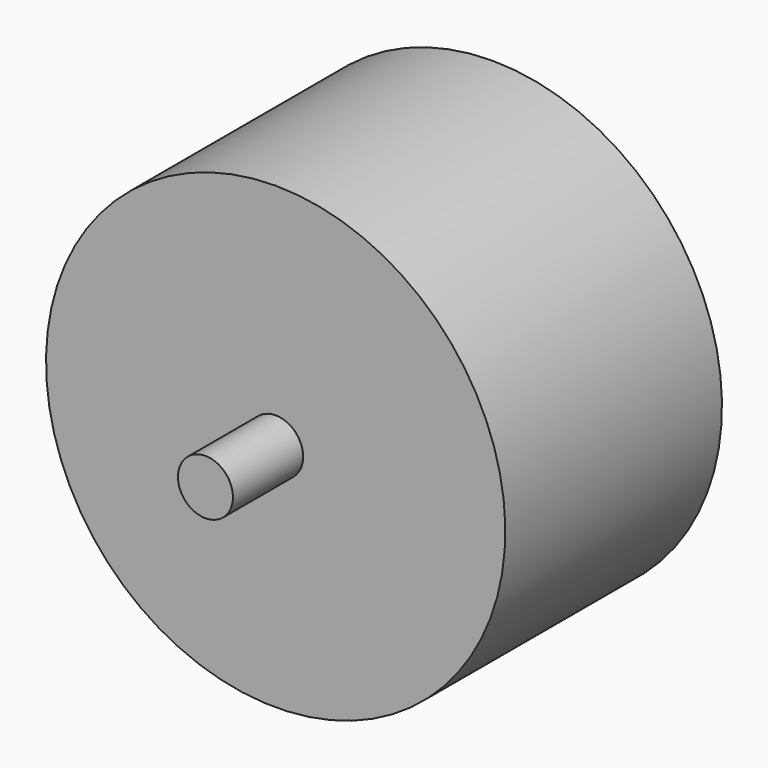
from build123d import *

# Parameters (mm, degrees)
F0_W         = 152.3266881704
F0_H         = 76.2925669551
F1_DEPTH     = 44.45
F2_T         = -2.54
F3_W         = 18.5941308737
F3_H         = 8.1849619746
F4_DEPTH     = 38.1
F5_T         = 2.54
F5_T3_DEPTH  = 13.2649619746
F5_T5_DEPTH  = 23.6741308737
F5_T7_DEPTH  = 78.8325669551
F5_T9_DEPTH  = 44.45
F5_T11_DEPTH = 152.3266881704
F7_R         = 5.6737308036
F8_DEPTH     = 89.211769402
F9_W         = 55.9205748141
F9_H         = 47.4143326283


# Not quite as in the source:
# - a shell that OpenCascade refuses in one call is made with other operations: the cavity is built on its own and cut out


with BuildPart() as f1:
    # F0 (on Front) → F1 (new body)
    with BuildSketch(Plane.XZ):
        with Locations((0.0222995877, 38.1462834775)):
            Rectangle(F0_W, F0_H)
    extrude(amount=F1_DEPTH)

    # F2
    f2_openings = [f1.faces().sort_by_distance(p)[0] for p in [
        (0.0223, -22.225, 0),
    ]]
    offset(amount=F2_T, openings=f2_openings)

    # F3 (on face) → F4 (join)
    with BuildSketch(Plane(origin=(-76.1410444975, 0, 0), x_dir=(0, -1, 0), z_dir=(-1, 0, 0))):
        with Locations((25.1720361412, 52.4518452585)):
            Rectangle(F3_W, F3_H)
    extrude(amount=F4_DEPTH)

    # F5: shell of thickness 2.54, made by hand


with BuildPart() as f5_core1:
    # F5_t2: copy of F1
    add(f1.part)

    # the walls: a layer under each face that stays
    f5_faces = [f5_core1.faces().sort_by_distance(p)[0] for p in [
        (0.0222995877, -22.225, 76.2925669551),
        (76.1856436729, -22.225, 38.1462834775),
        (-76.1410444975, -22.225, 38.1462834775),
        (0.0222995877, 0, 38.1462834775),
        (0.0222995877, -44.45, 38.1462834775),
        (-71.0634882251, -42.9683333333, 0),
        (-95.1910444975, -34.469101578, 52.4518452585),
        (-95.1910444975, -25.1720361412, 48.3593642712),
        (-95.1910444975, -15.8749707043, 52.4518452585),
        (-73.6010444975, -22.225, 36.8762834775),
        (0.0222995877, -2.54, 36.8762834775),
        (73.6456436729, -22.225, 36.8762834775),
        (0.0222995877, -41.91, 36.8762834775),
        (0.0222995877, -22.225, 73.7525669551),
    ]]
    thicken(f5_faces, amount=-F5_T, mode=Mode.SUBTRACT)

    # F5_s4 → F5_t3 (cut)
    with BuildSketch(Plane.XY.offset(45.8193642712)):
        Polygon((-76.1664444975, -34.494501578), (-73.6010444975, -34.469101578), (-73.6010444975, -31.929101578), (-76.1410444975, -31.929101578), align=None)
        Polygon((-76.1664444975, -15.8495707043), (-73.6010444975, -15.8749707043), (-73.6010444975, -18.4149707043), (-76.1410444975, -18.4149707043), align=None)
    extrude(amount=F5_T3_DEPTH, mode=Mode.SUBTRACT)

    # F5_s6 → F5_t5 (cut)
    with BuildSketch(Plane.XZ.offset(13.3349707043)):
        Polygon((-76.1664444975, 48.3339642712), (-73.6010444975, 48.3593642712), (-73.6010444975, 50.8993642712), (-76.1410444975, 50.8993642712), align=None)
    extrude(amount=F5_T5_DEPTH, mode=Mode.SUBTRACT)

    # F5_s8 → F5_t7 (cut)
    with BuildSketch(Plane.XY.offset(-2.54)):
        Polygon((-73.5756444975, -2.5654), (-76.1410444975, -2.54), (-76.1410444975, 0), (-73.6010444975, 0), align=None)
        Polygon((-73.5756444975, -41.8846), (-76.1410444975, -41.91), (-76.1410444975, -44.45), (-73.6010444975, -44.45), align=None)
        Polygon((73.6202436729, -2.5654), (73.6456436729, 0), (76.1856436729, 0), (76.1856436729, -2.54), align=None)
        Polygon((73.6202436729, -41.8846), (76.1856436729, -41.91), (76.1856436729, -44.45), (73.6456436729, -44.45), align=None)
    extrude(amount=F5_T7_DEPTH, mode=Mode.SUBTRACT)

    # F5_s10 → F5_t9 (cut)
    with BuildSketch(Plane.XZ):
        Polygon((-73.5756444975, 73.7271669551), (-76.1410444975, 73.7525669551), (-76.1410444975, 76.2925669551), (-73.6010444975, 76.2925669551), align=None)
        Polygon((73.6202436729, 73.7271669551), (76.1856436729, 73.7525669551), (76.1856436729, 76.2925669551), (73.6456436729, 76.2925669551), align=None)
    extrude(amount=F5_T9_DEPTH, mode=Mode.SUBTRACT)

    # F5_s12 → F5_t11 (cut)
    with BuildSketch(Plane.YZ.offset(-76.1410444975)):
        Polygon((-2.5654, 73.7271669551), (0, 73.7525669551), (0, 76.2925669551), (-2.54, 76.2925669551), align=None)
        Polygon((-41.8846, 73.7271669551), (-44.45, 73.7525669551), (-44.45, 76.2925669551), (-41.91, 76.2925669551), align=None)
    extrude(amount=F5_T11_DEPTH, mode=Mode.SUBTRACT)


with BuildPart() as f1_1:
    add(f1.part)

    # what is left inside the walls is the cavity
    f5_cavity = [f5_core1.part.solids().sort_by_distance(p)[0] for p in [
        (-101.541044, -25.172036, 56.518926),
    ]]
    add(f5_cavity, mode=Mode.SUBTRACT)


with BuildPart() as f8:
    # F7 (on Front) → F8 (new body)
    with BuildSketch(Plane.XZ):
        Circle(F7_R)
    extrude(amount=F8_DEPTH)

    # F9 (on Right) → F10 (revolve)
    with BuildSketch(Plane.YZ):
        with Locations((-43.1295465678, 23.7071663141)):
            Rectangle(F9_W, F9_H)
    revolve(axis=Axis((0, -43.1295465678, 0), (0, -1, 0)))


solid = f8.part
